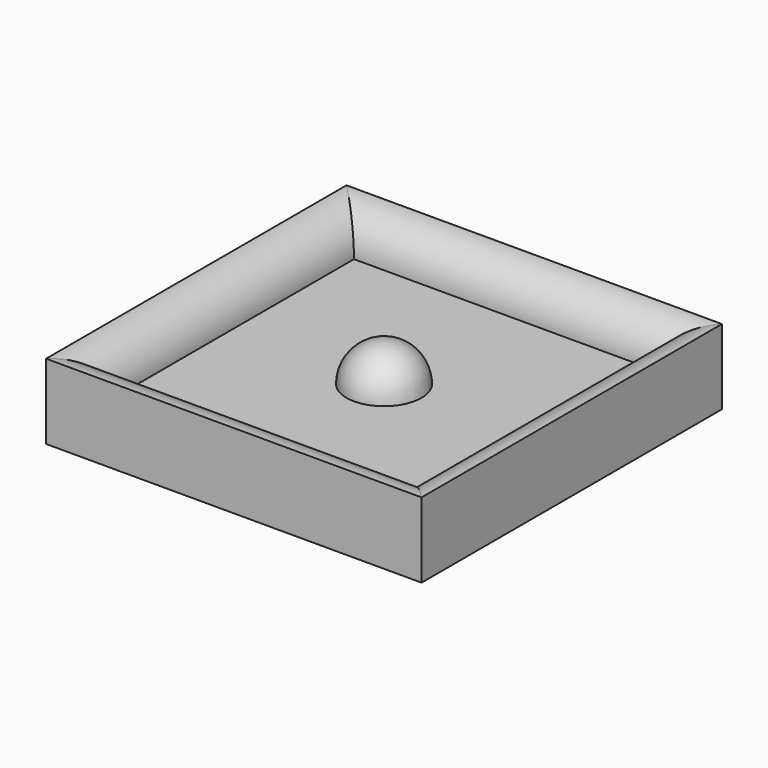
from build123d import *

# Parameters (mm, degrees)
F0_W     = 31.75
F0_H     = 31.75
F0_W_2   = 25.4
F0_H_2   = 25.4
F1_DEPTH = 3.175
F2_DEPTH = 6.35
F6_R     = 3.17499


# Not quite as in the source:
# - a fillet or chamfer is up to 0.001 mm smaller than in the source, because OpenCascade refuses the exact size


with BuildPart() as f1:
    # F0 (on Top) → F1 (new body)
    with BuildSketch(Plane.XY):
        Rectangle(F0_W, F0_H)
        Rectangle(F0_W_2, F0_H_2, mode=Mode.SUBTRACT)
        Rectangle(F0_W_2, F0_H_2)
        with BuildLine():
            ThreePointArc((0, 3.175), (2.2450640303, 2.2450640303), (3.175, 0))
            ThreePointArc((3.175, 0), (2.2450640303, -2.2450640303), (0, -3.175))
            ThreePointArc((0, -3.175), (-3.175, 0), (0, 3.175))
        make_face(mode=Mode.SUBTRACT)
        with BuildLine():
            ThreePointArc((0, -3.175), (2.2450640303, -2.2450640303), (3.175, 0))
            ThreePointArc((3.175, 0), (2.2450640303, 2.2450640303), (0, 3.175))
            Line((0, 3.175), (0, -3.175))
        make_face()
        with BuildLine():
            Line((0, -3.175), (0, 3.175))
            ThreePointArc((0, 3.175), (-3.175, 0), (0, -3.175))
        make_face()
    extrude(amount=F1_DEPTH)

    # F0 (on Top) → F2 (join)
    with BuildSketch(Plane.XY):
        Rectangle(F0_W, F0_H)
        Rectangle(F0_W_2, F0_H_2, mode=Mode.SUBTRACT)
    extrude(amount=F2_DEPTH)

    # F3 (on face) → F4 (revolve)
    with BuildSketch(Plane.XY.offset(3.175)):
        with BuildLine():
            Line((0, -3.175), (0, 3.175))
            ThreePointArc((0, 3.175), (-3.175, 0), (0, -3.175))
        make_face()
    revolve(axis=Axis((0, 0, 3.175), (0, 1, 0)))

    # F0 (on Top) → F5 (revolve, cut)
    with BuildSketch(Plane.XY):
        with BuildLine():
            Line((0, -3.175), (0, 3.175))
            ThreePointArc((0, 3.175), (-3.175, 0), (0, -3.175))
        make_face()
    revolve(axis=Axis((0, 0, 0), (0, 1, 0)), mode=Mode.SUBTRACT)

    # F6 (radius 3.175 in the source; OpenCascade refuses exactly that, so slightly less here)
    f6_edges = [f1.edges().sort_by_distance(p)[0] for p in [
        (0, 12.7, 6.35),
        (12.7, 0, 6.35),
        (-12.7, 0, 6.35),
        (0, -12.7, 6.35),
    ]]
    fillet(f6_edges, radius=F6_R)


solid = f1.part
